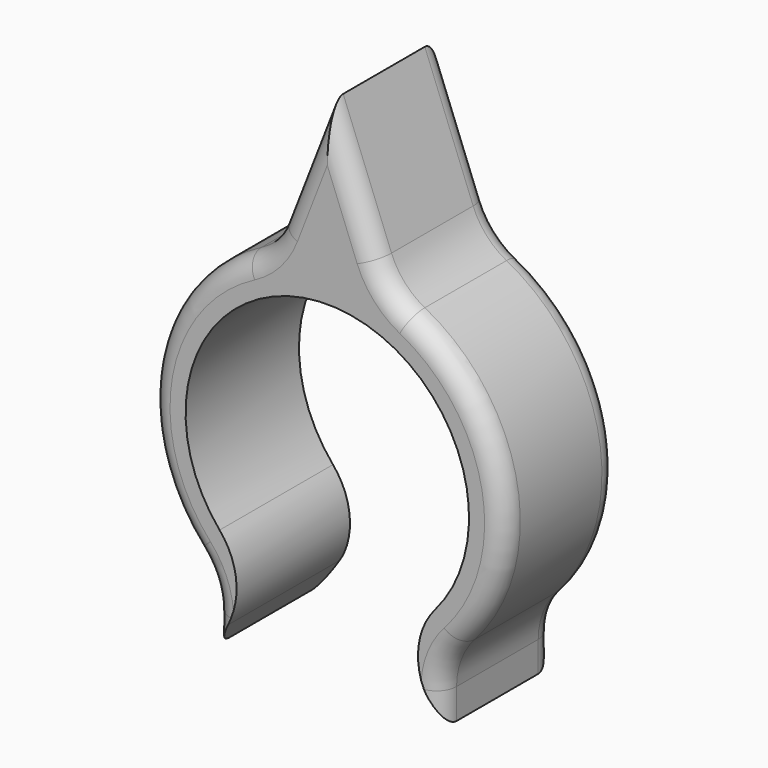
from build123d import *

# Parameters (mm, degrees)
F1_DEPTH     = 10
F2_R         = 5
F3_R         = 5
F4_R         = 5
F5_R         = 5
F6_R         = 5
F7_T1_DEPTH  = 12.9209860369
F7_T3_DEPTH  = 12.9209860369
F7_T5_DEPTH  = 5.6410319467
F7_T8_ANGLE  = 41.3143422779
F7_T10_ANGLE = 104.5599421702
F7_T12_ANGLE = 42.0246275794
F7_T14_ANGLE = 41.3143422779
F7_T16_ANGLE = 104.5599421702
F7_T18_ANGLE = 42.0246275794
F8_T1_DEPTH  = 12.9209860369
F8_T3_DEPTH  = 12.9209860369
F8_T5_DEPTH  = 5.6410319467
F8_T8_ANGLE  = 42.0246275794
F8_T10_ANGLE = 42.0246275794
F8_T12_ANGLE = 104.5599421702
F8_T14_ANGLE = 104.5599421702
F8_T16_ANGLE = 41.3143422779
F8_T18_ANGLE = 41.3143422779


# Not quite as in the source:
# - a fillet or chamfer that OpenCascade refuses, or shapes differently, is made with other operations: its cross-section is extruded or revolved along the edge and cut away or added


with BuildPart() as f1:
    # F0 (on Front) → F1 (new body)
    with BuildSketch(Plane.XZ):
        with BuildLine():
            ThreePointArc((-5, -8.6602540378), (0, 10), (5, -8.6602540378))
            Line((5, -8.6602540378), (6.25, -10.8253175473))
            Line((6.25, -10.8253175473), (8, -13.8564064606))
            Line((8, -13.8564064606), (8, -9.6046863561))
            ThreePointArc((8, -9.6046863561), (12.3033115605, 2.2087382474), (4.1595701998, 11.7876195965))
            ThreePointArc((4.1595701998, 11.7876195965), (0, 12.5), (-4.1595701998, 11.7876195965))
            ThreePointArc((-4.1595701998, 11.7876195965), (-12.3033115605, 2.2087382474), (-8, -9.6046863561))
            Line((-8, -9.6046863561), (-8, -13.8564064606))
            Line((-8, -13.8564064606), (-6.25, -10.8253175473))
            Line((-6.25, -10.8253175473), (-5, -8.6602540378))
        make_face()
        with BuildLine():
            ThreePointArc((-4.1595701998, 11.7876195965), (0, 12.5), (4.1595701998, 11.7876195965))
            Line((4.1595701998, 11.7876195965), (0, 22.5))
            Line((0, 22.5), (-4.1595701998, 11.7876195965))
        make_face()
    extrude(amount=F1_DEPTH)

    # F2
    f2_edges = [f1.edges().sort_by_distance(p)[0] for p in [
        (-4.15957, -5, 11.78762),
    ]]
    fillet(f2_edges, radius=F2_R)

    # F3
    f3_edges = [f1.edges().sort_by_distance(p)[0] for p in [
        (4.15957, -5, 11.78762),
    ]]
    fillet(f3_edges, radius=F3_R)

    # F4
    f4_edges = [f1.edges().sort_by_distance(p)[0] for p in [
        (-5, -5, -8.660254),
    ]]
    fillet(f4_edges, radius=F4_R)

    # F5
    f5_edges = [f1.edges().sort_by_distance(p)[0] for p in [
        (-8, -5, -9.604686),
    ]]
    fillet(f5_edges, radius=F5_R)

    # F6
    f6_edges = [f1.edges().sort_by_distance(p)[0] for p in [
        (8, -5, -9.604686),
        (5, -5, -8.660254),
    ]]
    fillet(f6_edges, radius=F6_R)

    # F7: fillet of radius 1.4 on 2 edges, made by hand

    # F7_s2 → F7_t1 (cut)
    with BuildSketch(Plane(origin=(-4.1819067631, 0, 10.7699050398), x_dir=(0, 1, 0), z_dir=(-0.3619658098, 0, 0.9321913712))):
        with BuildLine():
            ThreePointArc((-8.6, -8.1442307215), (-9.5899494937, -7.7341802151), (-10, -6.7442307215))
            Line((-10, -6.7442307215), (-10, -8.1442307215))
            Line((-10, -8.1442307215), (-8.6, -8.1442307215))
        make_face()
    extrude(amount=F7_T1_DEPTH, mode=Mode.SUBTRACT)

    # F7_s4 → F7_t3 (cut)
    with BuildSketch(Plane(origin=(8.8588619379, 0, 22.8147367305), x_dir=(0, 1, 0), z_dir=(-0.3619658098, 0, -0.9321913712))):
        with BuildLine():
            ThreePointArc((-8.6, -8.1442307215), (-9.5899494937, -7.7341802151), (-10, -6.7442307215))
            Line((-10, -6.7442307215), (-10, -8.1442307215))
            Line((-10, -8.1442307215), (-8.6, -8.1442307215))
        make_face()
    extrude(amount=F7_T3_DEPTH, mode=Mode.SUBTRACT)

    # F7_s6 → F7_t5 (cut)
    with BuildSketch(Plane.XY.offset(-17.3564064606)):
        with BuildLine():
            ThreePointArc((-8, -8.6), (-7.5899494937, -9.5899494937), (-6.6, -10))
            Line((-6.6, -10), (-8, -10))
            Line((-8, -10), (-8, -8.6))
        make_face()
        with BuildLine():
            ThreePointArc((8, -8.6), (7.5899494937, -9.5899494937), (6.6, -10))
            Line((6.6, -10), (8, -10))
            Line((8, -10), (8, -8.6))
        make_face()
    extrude(amount=F7_T5_DEPTH, mode=Mode.SUBTRACT)

    # F7_s7 → F7_t8 (revolve, cut)
    with BuildSketch(Plane(origin=(4.1819067631, 0, 10.7699050398), x_dir=(0, 1, 0), z_dir=(0.3619658098, 0, 0.9321913712))):
        with BuildLine():
            ThreePointArc((-8.6, 8.1442307215), (-9.5899494937, 7.7341802151), (-10, 6.7442307215))
            Line((-10, 6.7442307215), (-10, 8.1442307215))
            Line((-10, 8.1442307215), (-8.6, 8.1442307215))
        make_face()
    revolve(axis=Axis((-8.0710316963, -10, 15.5276671576), (0, 1, 0)), revolution_arc=F7_T8_ANGLE, mode=Mode.SUBTRACT)

    # F7_s9 → F7_t10 (revolve, cut)
    with BuildSketch(Plane(origin=(0, 0, 0), x_dir=(0, 1, 0), z_dir=(0.8872952661, 0, 0.4612018112))):
        with BuildLine():
            ThreePointArc((-8.6, 12.5), (-9.5899494937, 12.0899494937), (-10, 11.1))
            Line((-10, 11.1), (-10, 12.5))
            Line((-10, 12.5), (-8.6, 12.5))
        make_face()
    revolve(axis=Axis((0, -10, 0), (0, -1, 0)), revolution_arc=F7_T10_ANGLE, mode=Mode.SUBTRACT)

    # F7_s11 → F7_t12 (revolve, cut)
    with BuildSketch(Plane.XY.offset(-11.7153745139)):
        with BuildLine():
            ThreePointArc((-8, -8.6), (-7.5899494937, -9.5899494937), (-6.6, -10))
            Line((-6.6, -10), (-8, -10))
            Line((-8, -10), (-8, -8.6))
        make_face()
    revolve(axis=Axis((-13, -10, -11.7153745139), (0, -1, 0)), revolution_arc=F7_T12_ANGLE, mode=Mode.SUBTRACT)

    # F7_s13 → F7_t14 (revolve, cut)
    with BuildSketch(Plane(origin=(-4.1819067631, 0, 10.7699050398), x_dir=(0, 1, 0), z_dir=(-0.3619658098, 0, 0.9321913712))):
        with BuildLine():
            ThreePointArc((-8.6, -8.1442307215), (-9.5899494937, -7.7341802151), (-10, -6.7442307215))
            Line((-10, -6.7442307215), (-10, -8.1442307215))
            Line((-10, -8.1442307215), (-8.6, -8.1442307215))
        make_face()
    revolve(axis=Axis((8.0710316963, -10, 15.5276671576), (0, -1, 0)), revolution_arc=F7_T14_ANGLE, mode=Mode.SUBTRACT)

    # F7_s15 → F7_t16 (revolve, cut)
    with BuildSketch(Plane(origin=(0, 0, 0), x_dir=(0, 1, 0), z_dir=(-0.6694499722, 0, -0.7428571429))):
        with BuildLine():
            ThreePointArc((-8.6, 12.5), (-9.5899494937, 12.0899494937), (-10, 11.1))
            Line((-10, 11.1), (-10, 12.5))
            Line((-10, 12.5), (-8.6, 12.5))
        make_face()
    revolve(axis=Axis((0, -10, 0), (0, -1, 0)), revolution_arc=F7_T16_ANGLE, mode=Mode.SUBTRACT)

    # F7_s17 → F7_t18 (revolve, cut)
    with BuildSketch(Plane.XY.offset(-11.7153745139)):
        with BuildLine():
            ThreePointArc((8, -8.6), (7.5899494937, -9.5899494937), (6.6, -10))
            Line((6.6, -10), (8, -10))
            Line((8, -10), (8, -8.6))
        make_face()
    revolve(axis=Axis((13, -10, -11.7153745139), (0, 1, 0)), revolution_arc=F7_T18_ANGLE, mode=Mode.SUBTRACT)

    # F8: fillet of radius 1.4 on 8 edges, made by hand

    # F8_s2 → F8_t1 (cut)
    with BuildSketch(Plane(origin=(-4.1819067631, 0, 10.7699050398), x_dir=(0, 1, 0), z_dir=(-0.3619658098, 0, 0.9321913712))):
        with BuildLine():
            ThreePointArc((0, -6.7442307215), (-0.4100505063, -7.7341802151), (-1.4, -8.1442307215))
            Line((-1.4, -8.1442307215), (0, -8.1442307215))
            Line((0, -8.1442307215), (0, -6.7442307215))
        make_face()
    extrude(amount=F8_T1_DEPTH, mode=Mode.SUBTRACT)

    # F8_s4 → F8_t3 (cut)
    with BuildSketch(Plane(origin=(8.8588619379, 0, 22.8147367305), x_dir=(0, 1, 0), z_dir=(-0.3619658098, 0, -0.9321913712))):
        with BuildLine():
            ThreePointArc((0, -6.7442307215), (-0.4100505063, -7.7341802151), (-1.4, -8.1442307215))
            Line((-1.4, -8.1442307215), (0, -8.1442307215))
            Line((0, -8.1442307215), (0, -6.7442307215))
        make_face()
    extrude(amount=F8_T3_DEPTH, mode=Mode.SUBTRACT)

    # F8_s6 → F8_t5 (cut)
    with BuildSketch(Plane.XY.offset(-17.3564064606)):
        with BuildLine():
            ThreePointArc((-6.6, 0), (-7.5899494937, -0.4100505063), (-8, -1.4))
            Line((-8, -1.4), (-8, 0))
            Line((-8, 0), (-6.6, 0))
        make_face()
        with BuildLine():
            ThreePointArc((6.6, 0), (7.5899494937, -0.4100505063), (8, -1.4))
            Line((8, -1.4), (8, 0))
            Line((8, 0), (6.6, 0))
        make_face()
    extrude(amount=F8_T5_DEPTH, mode=Mode.SUBTRACT)

    # F8_s7 → F8_t8 (revolve, cut)
    with BuildSketch(Plane.XY.offset(-11.7153745139)):
        with BuildLine():
            ThreePointArc((6.6, 0), (7.5899494937, -0.4100505063), (8, -1.4))
            Line((8, -1.4), (8, 0))
            Line((8, 0), (6.6, 0))
        make_face()
    revolve(axis=Axis((13, 0, -11.7153745139), (0, 1, 0)), revolution_arc=F8_T8_ANGLE, mode=Mode.SUBTRACT)

    # F8_s9 → F8_t10 (revolve, cut)
    with BuildSketch(Plane.XY.offset(-11.7153745139)):
        with BuildLine():
            ThreePointArc((-6.6, 0), (-7.5899494937, -0.4100505063), (-8, -1.4))
            Line((-8, -1.4), (-8, 0))
            Line((-8, 0), (-6.6, 0))
        make_face()
    revolve(axis=Axis((-13, 0, -11.7153745139), (0, -1, 0)), revolution_arc=F8_T10_ANGLE, mode=Mode.SUBTRACT)

    # F8_s11 → F8_t12 (revolve, cut)
    with BuildSketch(Plane(origin=(0, 0, 0), x_dir=(0, 1, 0), z_dir=(-0.6694499722, 0, -0.7428571429))):
        with BuildLine():
            ThreePointArc((0, 11.1), (-0.4100505063, 12.0899494937), (-1.4, 12.5))
            Line((-1.4, 12.5), (0, 12.5))
            Line((0, 12.5), (0, 11.1))
        make_face()
    revolve(axis=Axis((0, 0, 0), (0, -1, 0)), revolution_arc=F8_T12_ANGLE, mode=Mode.SUBTRACT)

    # F8_s13 → F8_t14 (revolve, cut)
    with BuildSketch(Plane(origin=(0, 0, 0), x_dir=(0, 1, 0), z_dir=(0.8872952661, 0, 0.4612018112))):
        with BuildLine():
            ThreePointArc((0, 11.1), (-0.4100505063, 12.0899494937), (-1.4, 12.5))
            Line((-1.4, 12.5), (0, 12.5))
            Line((0, 12.5), (0, 11.1))
        make_face()
    revolve(axis=Axis((0, 0, 0), (0, -1, 0)), revolution_arc=F8_T14_ANGLE, mode=Mode.SUBTRACT)

    # F8_s15 → F8_t16 (revolve, cut)
    with BuildSketch(Plane(origin=(-4.1819067631, 0, 10.7699050398), x_dir=(0, 1, 0), z_dir=(-0.3619658098, 0, 0.9321913712))):
        with BuildLine():
            ThreePointArc((0, -6.7442307215), (-0.4100505063, -7.7341802151), (-1.4, -8.1442307215))
            Line((-1.4, -8.1442307215), (0, -8.1442307215))
            Line((0, -8.1442307215), (0, -6.7442307215))
        make_face()
    revolve(axis=Axis((8.0710316963, 0, 15.5276671576), (0, -1, 0)), revolution_arc=F8_T16_ANGLE, mode=Mode.SUBTRACT)

    # F8_s17 → F8_t18 (revolve, cut)
    with BuildSketch(Plane(origin=(4.1819067631, 0, 10.7699050398), x_dir=(0, 1, 0), z_dir=(0.3619658098, 0, 0.9321913712))):
        with BuildLine():
            ThreePointArc((0, 6.7442307215), (-0.4100505063, 7.7341802151), (-1.4, 8.1442307215))
            Line((-1.4, 8.1442307215), (0, 8.1442307215))
            Line((0, 8.1442307215), (0, 6.7442307215))
        make_face()
    revolve(axis=Axis((-8.0710316963, 0, 15.5276671576), (0, 1, 0)), revolution_arc=F8_T18_ANGLE, mode=Mode.SUBTRACT)


solid = f1.part
